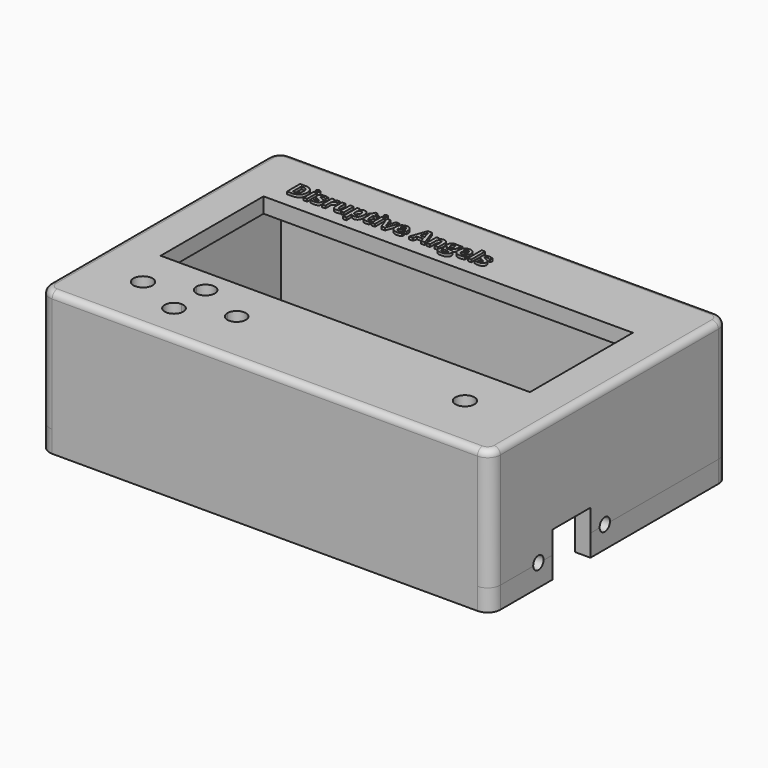
from build123d import *

# Parameters (mm, degrees)
F0_W         = 89.916
F0_H         = 59.436
F0_W_2       = 83.82
F0_H_2       = 53.34
F1_DEPTH     = 3.048
F2_DEPTH     = 17.78
F3_W         = 89.916
F3_H         = 59.436
F3_W_2       = 83.82
F3_H_2       = 53.34
F3_W_3       = 73.66
F3_H_3       = 25.654
F4_DEPTH     = 3.048
F5_TEXT_SIZE = 4.5443108926
F6_DEPTH     = 0.508
F7_DEPTH     = 3.302
F8_DEPTH     = 3.302
F9_R         = 2.54
F10_DEPTH    = 4.318
F11_R        = 1.27
F12_W        = 9.4091603532
F12_H        = 8.7967784599
F13_DEPTH    = 254
F12_R        = 1.2879927822
F12_R_2      = 1.2890101332
F14_DEPTH    = 279.4
F15_R        = 1.905
F16_DEPTH    = 25.4


# Not quite as in the source:
# - Text() gives the source's letters only with a copy of the font that has no kerning and outlines rounded to 1/6400 em; it was checked with that copy


with BuildPart() as f1:
    # F0 (on Top) → F1 (new body)
    with BuildSketch(Plane.XY):
        with Locations((-44.958, 29.718)):
            Rectangle(F0_W, F0_H)
        with Locations((-44.958, 29.718)):
            Rectangle(F0_W_2, F0_H_2, mode=Mode.SUBTRACT)
        with Locations((-44.958, 29.718)):
            Rectangle(F0_W_2, F0_H_2)
    extrude(amount=F1_DEPTH)

    # F0 (on Top) → F2 (join)
    with BuildSketch(Plane.XY):
        with Locations((-44.958, 29.718)):
            Rectangle(F0_W, F0_H)
        with Locations((-44.958, 29.718)):
            Rectangle(F0_W_2, F0_H_2, mode=Mode.SUBTRACT)
    extrude(amount=F2_DEPTH)

    # F3 (on face) → F4 (join)
    with BuildSketch(Plane.XY.offset(17.78)):
        with Locations((-44.958, 29.718)):
            Rectangle(F3_W, F3_H)
        with Locations((-44.958, 29.718)):
            Rectangle(F3_W_2, F3_H_2, mode=Mode.SUBTRACT)
        with Locations((-44.958, 29.718)):
            Rectangle(F3_W_2, F3_H_2)
        with Locations((-44.958, 32.893)):
            Rectangle(F3_W_3, F3_H_3, mode=Mode.SUBTRACT)
    extrude(amount=F4_DEPTH)

    # F5 (on face) → F6 (join)
    with BuildSketch(Plane.XY.offset(20.828)):
        with Locations((-79.756, 48.5440961573)):
            Text('Disruptive Angels', F5_TEXT_SIZE, font='Open Sans', font_style=FontStyle.BOLD, text_align=(TextAlign.LEFT, TextAlign.BOTTOM))
    extrude(amount=F6_DEPTH)

    # F0 (on Top) → F7 (cut)
    with BuildSketch(Plane.XY):
        with Locations((-44.958, 29.718)):
            Rectangle(F0_W, F0_H)
        with Locations((-44.958, 29.718)):
            Rectangle(F0_W_2, F0_H_2, mode=Mode.SUBTRACT)
        with Locations((-44.958, 29.718)):
            Rectangle(F0_W_2, F0_H_2)
    extrude(amount=F7_DEPTH, mode=Mode.SUBTRACT)

    # F0 (on Top) → F8 (join, symmetric)
    with BuildSketch(Plane.XY):
        with Locations((-44.958, 29.718)):
            Rectangle(F0_W, F0_H)
        with Locations((-44.958, 29.718)):
            Rectangle(F0_W_2, F0_H_2, mode=Mode.SUBTRACT)
    extrude(amount=F8_DEPTH, both=True)

    # F9
    f9_edges = [f1.edges().sort_by_distance(p)[0] for p in [
        (0, 0, 8.763),
        (0, 59.436, 8.763),
        (-89.916, 59.436, 8.763),
        (-89.916, 0, 8.763),
    ]]
    fillet(f9_edges, radius=F9_R)

    # F10 (add): a face of the model
    f10_faces = [f1.faces().sort_by_distance(p)[0] for p in [
        (-44.958, 1.0778462391, -3.302),
    ]]
    extrude(f10_faces, amount=F10_DEPTH)

    # F11
    f11_edges = [f1.edges().sort_by_distance(p)[0] for p in [
        (-44.958, 0, 20.828),
    ]]
    fillet(f11_edges, radius=F11_R)

    # F12 (on face) → F13 (cut)
    with BuildSketch(Plane(origin=(-89.916, 0, 0), x_dir=(0, -1, 0), z_dir=(-1, 0, 0))):
        with Locations((-20.2903314494, -3.22161077)):
            Rectangle(F12_W, F12_H)
    extrude(amount=-F13_DEPTH, mode=Mode.SUBTRACT)

    # F12 (on face) → F14 (cut)
    with BuildSketch(Plane(origin=(-89.916, 0, 0), x_dir=(0, -1, 0), z_dir=(-1, 0, 0))):
        with Locations((-28.577959165, -3.22161077)):
            Circle(F12_R)
        with Locations((-12.0157049969, -3.22161077)):
            Circle(F12_R_2)
    extrude(amount=-F14_DEPTH, mode=Mode.SUBTRACT)

    # F15 (on face) → F16 (cut)
    with BuildSketch(Plane.XY.offset(20.828)):
        with BuildLine():
            ThreePointArc((-69.0914208396, 13.5519117014), (-67.7856235995, 14.092790628), (-67.244744673, 15.3985878681))
            ThreePointArc((-67.244744673, 15.3985878681), (-69.0914208396, 17.2452640347), (-70.9380970063, 15.3985878681))
            ThreePointArc((-70.9380970063, 15.3985878681), (-70.3972180797, 14.092790628), (-69.0914208396, 13.5519117014))
        make_face()
        with BuildLine():
            ThreePointArc((-12.3009541715, 11.4599914971), (-14.2014315352, 13.3604688607), (-16.1019088988, 11.4599914971))
            ThreePointArc((-16.1019088988, 11.4599914971), (-14.2014315352, 9.5595141334), (-12.3009541715, 11.4599914971))
        make_face()
        with BuildLine():
            ThreePointArc((-57.9015623938, 11.4599914971), (-59.7484693299, 13.3068984332), (-61.595376266, 11.4599914971))
            ThreePointArc((-61.595376266, 11.4599914971), (-59.7484693299, 9.6130845609), (-57.9015623938, 11.4599914971))
        make_face()
        with BuildLine():
            ThreePointArc((-67.2385205879, 7.5213951261), (-67.7812225068, 8.8315934589), (-69.0914208396, 9.3742953778))
            ThreePointArc((-69.0914208396, 9.3742953778), (-70.4016191725, 6.2111967932), (-67.2385205879, 7.5213951261))
        make_face()
        with Locations((-78.4188931186, 11.4599914971)):
            Circle(F15_R)
    extrude(amount=-F16_DEPTH, mode=Mode.SUBTRACT)


solid = f1.part
